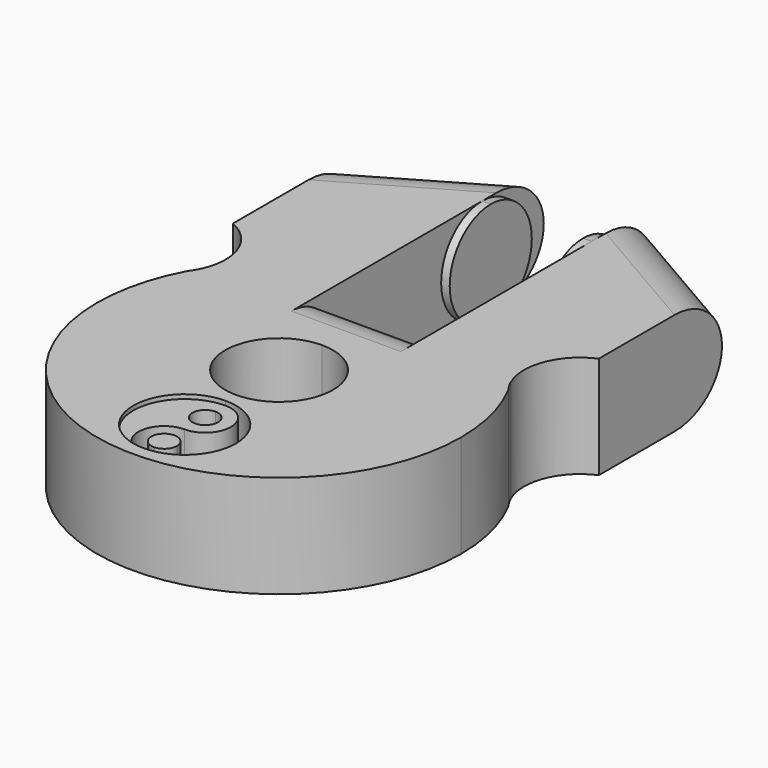
from build123d import *

# Parameters (mm, degrees)
F1_DEPTH  = 6
F3_DEPTH  = 0.5
F5_DEPTH  = 0.5
F6_R      = 2.99999
F7_R      = 2.99999
F9_DEPTH  = 2
F10_DEPTH = 0.25
F11_R     = 0.75
F12_DEPTH = 2
F13_DEPTH = 0.25


# Not quite as in the source:
# - a fillet or chamfer is up to 0.001 mm smaller than in the source, because OpenCascade refuses the exact size


with BuildPart() as f1:
    # F0 (on Top) → F1 (new body)
    with BuildSketch(Plane.XY):
        with BuildLine():
            ThreePointArc((-21.257927263, 3.0925971456), (-19.5135237331, 1.2849088277), (-19.5663380414, -1.2266427602))
            ThreePointArc((-19.5663380414, -1.2266427602), (-17.0596555887, 1.5276447909), (-13.757927263, 3.2504758611))
            Line((-13.757927263, 3.2504758611), (-13.757927263, 16.4425971456))
            Line((-13.757927263, 16.4425971456), (-21.257927263, 12.0925971456))
            Line((-21.257927263, 12.0925971456), (-21.257927263, 3.0925971456))
        make_face()
        with BuildLine():
            ThreePointArc((-19.937029438, -1.8621137259), (-13.1593751133, -17.2347921219), (0.092072737, -6.9074028544))
            ThreePointArc((0.092072737, -6.9074028544), (-0.2305379955, -4.3059550041), (-1.178825088, -1.8621137259))
            ThreePointArc((-1.178825088, -1.8621137259), (-1.3821012217, -1.5548376637), (-1.5495164847, -1.2266427602))
            ThreePointArc((-1.5495164847, -1.2266427602), (-4.0561989374, 1.5276447909), (-7.357927263, 3.2504758611))
            Line((-7.357927263, 3.2504758611), (-7.357927263, 1.1925971456))
            Line((-7.357927263, 1.1925971456), (-7.357927263, 0.9928541258))
            Line((-7.357927263, 0.9928541258), (-10.557927263, 0.9928541258))
            Line((-10.557927263, 0.9928541258), (-13.757927263, 0.9928541258))
            Line((-13.757927263, 0.9928541258), (-13.757927263, 1.1925971456))
            Line((-13.757927263, 1.1925971456), (-13.757927263, 3.2504758611))
            ThreePointArc((-13.757927263, 3.2504758611), (-17.0596555887, 1.5276447909), (-19.5663380414, -1.2266427602))
            ThreePointArc((-19.5663380414, -1.2266427602), (-19.7337533043, -1.5548376637), (-19.937029438, -1.8621137259))
        make_face()
        with BuildLine():
            ThreePointArc((-7.407927263, -6.9074028544), (-12.7853136237, -9.1347892152), (-10.557927263, -3.7574028544))
            ThreePointArc((-10.557927263, -3.7574028544), (-8.3305409023, -4.6800164937), (-7.407927263, -6.9074028544))
        make_face(mode=Mode.SUBTRACT)
        with BuildLine():
            ThreePointArc((-7.357927263, 3.2504758611), (-4.0561989374, 1.5276447909), (-1.5495164847, -1.2266427602))
            ThreePointArc((-1.5495164847, -1.2266427602), (-1.6023307929, 1.2849088277), (0.142072737, 3.0925971456))
            Line((0.142072737, 3.0925971456), (0.142072737, 12.0925971456))
            Line((0.142072737, 12.0925971456), (-7.357927263, 16.4425971456))
            Line((-7.357927263, 16.4425971456), (-7.357927263, 3.2504758611))
        make_face()
    extrude(amount=F1_DEPTH)

    # F2 (on face) → F3 (join)
    with BuildSketch(Plane.YZ.offset(-13.757927263)):
        with BuildLine():
            ThreePointArc((11.9425971456, 0), (14.0639174891, 0.8786796564), (14.9425971456, 3))
            ThreePointArc((14.9425971456, 3), (14.0639174891, 5.1213203436), (11.9425971456, 6))
            ThreePointArc((11.9425971456, 6), (8.9425971456, 3), (11.9425971456, 0))
        make_face()
    extrude(amount=F3_DEPTH)

    # F4 (on face) → F5 (join)
    with BuildSketch(Plane(origin=(-7.357927263, 0, 0), x_dir=(0, -1, 0), z_dir=(-1, 0, 0))):
        with BuildLine():
            ThreePointArc((-11.9425971456, 0), (-9.821276802, 0.8786796564), (-8.9425971456, 3))
            ThreePointArc((-8.9425971456, 3), (-9.821276802, 5.1213203436), (-11.9425971456, 6))
            ThreePointArc((-11.9425971456, 6), (-14.9425971456, 3), (-11.9425971456, 0))
        make_face()
    extrude(amount=F5_DEPTH)

    # F6 (radius 3 in the source; OpenCascade refuses exactly that, so slightly less here)
    f6_edges = [f1.edges().sort_by_distance(p)[0] for p in [
        (-10.557927, 0.992854, 0),
        (-10.557927, 0.992854, 6),
    ]]
    fillet(f6_edges, radius=F6_R)

    # F7 (radius 3 in the source; OpenCascade refuses exactly that, so slightly less here)
    f7_edges = [f1.edges().sort_by_distance(p)[0] for p in [
        (-3.607927, 14.267597, 6),
        (-3.607927, 14.267597, 0),
        (-17.507927, 14.267597, 6),
        (-17.507927, 14.267597, 0),
    ]]
    fillet(f7_edges, radius=F7_R)

    # F8 (on face) → F9 (cut)
    with BuildSketch(Plane.XY.offset(6)):
        with BuildLine():
            ThreePointArc((-10.557927263, -13.8074028544), (-12.057927263, -15.3074028544), (-10.557927263, -16.8074028544))
            Line((-10.557927263, -16.8074028544), (-10.557927263, -16.0574028544))
            ThreePointArc((-10.557927263, -16.0574028544), (-11.307927263, -15.3074028544), (-10.557927263, -14.5574028544))
            Line((-10.557927263, -14.5574028544), (-10.557927263, -13.8074028544))
        make_face()
        with BuildLine():
            ThreePointArc((-7.557927263, -13.8074028544), (-8.4366069195, -11.6860825109), (-10.557927263, -10.8074028544))
            ThreePointArc((-10.557927263, -10.8074028544), (-9.057927263, -12.3074028544), (-10.557927263, -13.8074028544))
            Line((-10.557927263, -13.8074028544), (-10.557927263, -14.5574028544))
            ThreePointArc((-10.557927263, -14.5574028544), (-10.0275971771, -14.7770727685), (-9.807927263, -15.3074028544))
            ThreePointArc((-9.807927263, -15.3074028544), (-10.0275971771, -15.8377329403), (-10.557927263, -16.0574028544))
            Line((-10.557927263, -16.0574028544), (-10.557927263, -16.8074028544))
            ThreePointArc((-10.557927263, -16.8074028544), (-8.4366069195, -15.928723198), (-7.557927263, -13.8074028544))
        make_face()
        with BuildLine():
            Line((-10.557927263, -13.0574028544), (-10.557927263, -11.5574028544))
            ThreePointArc((-10.557927263, -11.5574028544), (-11.307927263, -12.3074028544), (-10.557927263, -13.0574028544))
        make_face()
        with BuildLine():
            ThreePointArc((-9.807927263, -12.3074028544), (-10.0275971771, -11.7770727685), (-10.557927263, -11.5574028544))
            Line((-10.557927263, -11.5574028544), (-10.557927263, -13.0574028544))
            ThreePointArc((-10.557927263, -13.0574028544), (-10.0275971771, -12.8377329403), (-9.807927263, -12.3074028544))
        make_face()
    extrude(amount=-F9_DEPTH, mode=Mode.SUBTRACT)

    # F8 (on face) → F10 (cut)
    with BuildSketch(Plane.XY.offset(6)):
        with BuildLine():
            Line((-10.557927263, -11.5574028544), (-10.557927263, -10.8074028544))
            ThreePointArc((-10.557927263, -10.8074028544), (-13.557927263, -13.8074028544), (-10.557927263, -16.8074028544))
            ThreePointArc((-10.557927263, -16.8074028544), (-12.057927263, -15.3074028544), (-10.557927263, -13.8074028544))
            Line((-10.557927263, -13.8074028544), (-10.557927263, -13.0574028544))
            ThreePointArc((-10.557927263, -13.0574028544), (-11.307927263, -12.3074028544), (-10.557927263, -11.5574028544))
        make_face()
        with BuildLine():
            ThreePointArc((-10.557927263, -13.8074028544), (-9.057927263, -12.3074028544), (-10.557927263, -10.8074028544))
            Line((-10.557927263, -10.8074028544), (-10.557927263, -11.5574028544))
            ThreePointArc((-10.557927263, -11.5574028544), (-10.0275971771, -11.7770727685), (-9.807927263, -12.3074028544))
            ThreePointArc((-9.807927263, -12.3074028544), (-10.0275971771, -12.8377329403), (-10.557927263, -13.0574028544))
            Line((-10.557927263, -13.0574028544), (-10.557927263, -13.8074028544))
        make_face()
        with BuildLine():
            Line((-10.557927263, -14.5574028544), (-10.557927263, -16.0574028544))
            ThreePointArc((-10.557927263, -16.0574028544), (-10.0275971771, -15.8377329403), (-9.807927263, -15.3074028544))
            ThreePointArc((-9.807927263, -15.3074028544), (-10.0275971771, -14.7770727685), (-10.557927263, -14.5574028544))
        make_face()
        with BuildLine():
            ThreePointArc((-10.557927263, -14.5574028544), (-11.307927263, -15.3074028544), (-10.557927263, -16.0574028544))
            Line((-10.557927263, -16.0574028544), (-10.557927263, -14.5574028544))
        make_face()
    extrude(amount=-F10_DEPTH, mode=Mode.SUBTRACT)

    # F11 (on face) → F12 (cut)
    with BuildSketch(Plane(origin=(0, 0, 0), x_dir=(1, 0, 0), z_dir=(0, 0, -1))):
        with BuildLine():
            ThreePointArc((-10.557927263, 13.8074028544), (-12.057927263, 15.3074028544), (-10.557927263, 16.8074028544))
            ThreePointArc((-10.557927263, 16.8074028544), (-13.557927263, 13.8074028544), (-10.557927263, 10.8074028544))
            ThreePointArc((-10.557927263, 10.8074028544), (-9.057927263, 12.3074028544), (-10.557927263, 13.8074028544))
        make_face()
        with Locations((-10.557927263, 12.3074028544)):
            Circle(F11_R, mode=Mode.SUBTRACT)
        with Locations((-10.557927263, 15.3074028544)):
            Circle(F11_R)
    extrude(amount=-F12_DEPTH, mode=Mode.SUBTRACT)

    # F11 (on face) → F13 (cut)
    with BuildSketch(Plane(origin=(0, 0, 0), x_dir=(1, 0, 0), z_dir=(0, 0, -1))):
        with BuildLine():
            ThreePointArc((-10.557927263, 10.8074028544), (-8.4366069195, 11.6860825109), (-7.557927263, 13.8074028544))
            ThreePointArc((-7.557927263, 13.8074028544), (-8.4366069195, 15.928723198), (-10.557927263, 16.8074028544))
            ThreePointArc((-10.557927263, 16.8074028544), (-12.057927263, 15.3074028544), (-10.557927263, 13.8074028544))
            ThreePointArc((-10.557927263, 13.8074028544), (-9.057927263, 12.3074028544), (-10.557927263, 10.8074028544))
        make_face()
        with Locations((-10.557927263, 15.3074028544)):
            Circle(F11_R, mode=Mode.SUBTRACT)
        with Locations((-10.557927263, 12.3074028544)):
            Circle(F11_R)
    extrude(amount=-F13_DEPTH, mode=Mode.SUBTRACT)


solid = f1.part
